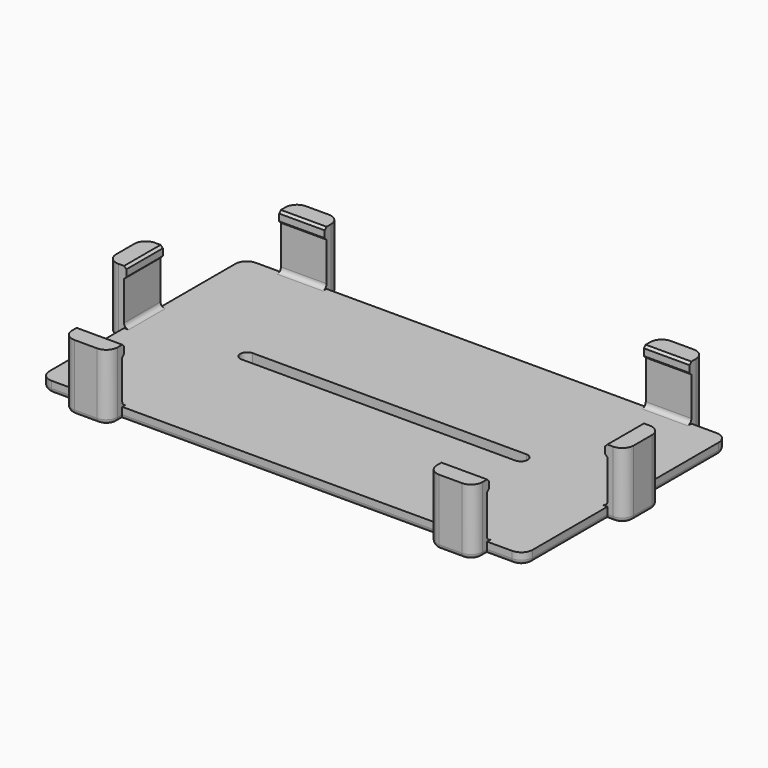
from build123d import *

# Parameters (mm, degrees)
F1_DEPTH = 3.175
F3_DEPTH = 15.24
F4_W     = 1.27
F4_H     = 12.7
F4_W_2   = 12.7
F4_H_2   = 1.27
F5_DEPTH = 3.175
F6_SIZE  = 1.26999
F8_W     = 133.35
F8_H     = 69.85
F9_DEPTH = 6.35
F10_R    = 1.27
F11_R    = 1.27


# Not quite as in the source:
# - a fillet or chamfer is up to 0.001 mm smaller than in the source, because OpenCascade refuses the exact size


with BuildPart() as f1:
    # F0 (on Top) → F1 (new body)
    with BuildSketch(Plane.XY):
        with BuildLine():
            ThreePointArc((67.31, 32.385), (66.3800640303, 34.6300640303), (64.135, 35.56))
            Line((64.135, 35.56), (-64.135, 35.56))
            ThreePointArc((-64.135, 35.56), (-66.3800640303, 34.6300640303), (-67.31, 32.385))
            Line((-67.31, 32.385), (-67.31, -32.385))
            ThreePointArc((-67.31, -32.385), (-66.3800640303, -34.6300640303), (-64.135, -35.56))
            Line((-64.135, -35.56), (64.135, -35.56))
            ThreePointArc((64.135, -35.56), (66.3800640303, -34.6300640303), (67.31, -32.385))
            Line((67.31, -32.385), (67.31, 32.385))
        make_face()
        with BuildLine():
            Line((38.1, -1.905), (-38.1, -1.905))
            ThreePointArc((-38.1, -1.905), (-40.005, 0), (-38.1, 1.905))
            Line((-38.1, 1.905), (38.1, 1.905))
            ThreePointArc((38.1, 1.905), (40.005, 0), (38.1, -1.905))
        make_face(mode=Mode.SUBTRACT)
    extrude(amount=F1_DEPTH)

    # F2 (on Top) → F3 (join)
    with BuildSketch(Plane.XY):
        with BuildLine():
            Line((-67.31, -6.35), (-67.31, 6.35))
            Line((-67.31, 6.35), (-68.8975, 6.35))
            ThreePointArc((-68.8975, 6.35), (-71.1425640303, 5.4200640303), (-72.0725, 3.175))
            Line((-72.0725, 3.175), (-72.0725, -3.175))
            ThreePointArc((-72.0725, -3.175), (-71.1425640303, -5.4200640303), (-68.8975, -6.35))
            Line((-68.8975, -6.35), (-67.31, -6.35))
        make_face()
        with BuildLine():
            Line((-44.45, -37.1475), (-44.45, -35.56))
            Line((-44.45, -35.56), (-57.15, -35.56))
            Line((-57.15, -35.56), (-57.15, -37.1475))
            ThreePointArc((-57.15, -37.1475), (-56.2200640303, -39.3925640303), (-53.975, -40.3225))
            Line((-53.975, -40.3225), (-47.625, -40.3225))
            ThreePointArc((-47.625, -40.3225), (-45.3799359697, -39.3925640303), (-44.45, -37.1475))
        make_face()
        with BuildLine():
            Line((-57.15, 35.56), (-44.45, 35.56))
            Line((-44.45, 35.56), (-44.45, 37.1475))
            ThreePointArc((-44.45, 37.1475), (-45.3799359697, 39.3925640303), (-47.625, 40.3225))
            Line((-47.625, 40.3225), (-53.975, 40.3225))
            ThreePointArc((-53.975, 40.3225), (-56.2200640303, 39.3925640303), (-57.15, 37.1475))
            Line((-57.15, 37.1475), (-57.15, 35.56))
        make_face()
        with BuildLine():
            Line((57.15, -35.56), (44.45, -35.56))
            Line((44.45, -35.56), (44.45, -37.1475))
            ThreePointArc((44.45, -37.1475), (45.3799359697, -39.3925640303), (47.625, -40.3225))
            Line((47.625, -40.3225), (53.975, -40.3225))
            ThreePointArc((53.975, -40.3225), (56.2200640303, -39.3925640303), (57.15, -37.1475))
            Line((57.15, -37.1475), (57.15, -35.56))
        make_face()
        with BuildLine():
            Line((67.31, 6.35), (67.31, -6.35))
            Line((67.31, -6.35), (68.8975, -6.35))
            ThreePointArc((68.8975, -6.35), (71.1425640303, -5.4200640303), (72.0725, -3.175))
            Line((72.0725, -3.175), (72.0725, 3.175))
            ThreePointArc((72.0725, 3.175), (71.1425640303, 5.4200640303), (68.8975, 6.35))
            Line((68.8975, 6.35), (67.31, 6.35))
        make_face()
        with BuildLine():
            Line((44.45, 35.56), (57.15, 35.56))
            Line((57.15, 35.56), (57.15, 37.1475))
            ThreePointArc((57.15, 37.1475), (56.2200640303, 39.3925640303), (53.975, 40.3225))
            Line((53.975, 40.3225), (47.625, 40.3225))
            ThreePointArc((47.625, 40.3225), (45.3799359697, 39.3925640303), (44.45, 37.1475))
            Line((44.45, 37.1475), (44.45, 35.56))
        make_face()
    extrude(amount=F3_DEPTH)

    # F4 (on face) → F5 (join)
    with BuildSketch(Plane.XY.offset(15.24)):
        with BuildLine():
            Line((-68.8975, -6.35), (-67.31, -6.35))
            Line((-67.31, -6.35), (-67.31, 6.35))
            Line((-67.31, 6.35), (-68.8975, 6.35))
            ThreePointArc((-68.8975, 6.35), (-71.1425640303, 5.4200640303), (-72.0725, 3.175))
            Line((-72.0725, 3.175), (-72.0725, -3.175))
            ThreePointArc((-72.0725, -3.175), (-71.1425640303, -5.4200640303), (-68.8975, -6.35))
        make_face()
        with Locations((-66.675, 0)):
            Rectangle(F4_W, F4_H)
        with BuildLine():
            Line((-44.45, -35.56), (-57.15, -35.56))
            Line((-57.15, -35.56), (-57.15, -37.1475))
            ThreePointArc((-57.15, -37.1475), (-56.2200640303, -39.3925640303), (-53.975, -40.3225))
            Line((-53.975, -40.3225), (-47.625, -40.3225))
            ThreePointArc((-47.625, -40.3225), (-45.3799359697, -39.3925640303), (-44.45, -37.1475))
            Line((-44.45, -37.1475), (-44.45, -35.56))
        make_face()
        with Locations((-50.8, -34.925)):
            Rectangle(F4_W_2, F4_H_2)
        with BuildLine():
            Line((-57.15, 37.1475), (-57.15, 35.56))
            Line((-57.15, 35.56), (-44.45, 35.56))
            Line((-44.45, 35.56), (-44.45, 37.1475))
            ThreePointArc((-44.45, 37.1475), (-45.3799359697, 39.3925640303), (-47.625, 40.3225))
            Line((-47.625, 40.3225), (-53.975, 40.3225))
            ThreePointArc((-53.975, 40.3225), (-56.2200640303, 39.3925640303), (-57.15, 37.1475))
        make_face()
        with Locations((-50.8, 34.925)):
            Rectangle(F4_W_2, F4_H_2)
        with Locations((50.8, 34.925)):
            Rectangle(F4_W_2, F4_H_2)
        with BuildLine():
            Line((44.45, 35.56), (57.15, 35.56))
            Line((57.15, 35.56), (57.15, 37.1475))
            ThreePointArc((57.15, 37.1475), (56.2200640303, 39.3925640303), (53.975, 40.3225))
            Line((53.975, 40.3225), (47.625, 40.3225))
            ThreePointArc((47.625, 40.3225), (45.3799359697, 39.3925640303), (44.45, 37.1475))
            Line((44.45, 37.1475), (44.45, 35.56))
        make_face()
        with Locations((66.675, 0)):
            Rectangle(F4_W, F4_H)
        with BuildLine():
            Line((68.8975, 6.35), (67.31, 6.35))
            Line((67.31, 6.35), (67.31, -6.35))
            Line((67.31, -6.35), (68.8975, -6.35))
            ThreePointArc((68.8975, -6.35), (71.1425640303, -5.4200640303), (72.0725, -3.175))
            Line((72.0725, -3.175), (72.0725, 3.175))
            ThreePointArc((72.0725, 3.175), (71.1425640303, 5.4200640303), (68.8975, 6.35))
        make_face()
        with BuildLine():
            Line((57.15, -37.1475), (57.15, -35.56))
            Line((57.15, -35.56), (44.45, -35.56))
            Line((44.45, -35.56), (44.45, -37.1475))
            ThreePointArc((44.45, -37.1475), (45.3799359697, -39.3925640303), (47.625, -40.3225))
            Line((47.625, -40.3225), (53.975, -40.3225))
            ThreePointArc((53.975, -40.3225), (56.2200640303, -39.3925640303), (57.15, -37.1475))
        make_face()
        with Locations((50.8, -34.925)):
            Rectangle(F4_W_2, F4_H_2)
    extrude(amount=F5_DEPTH)

    # F6 (size 1.27 in the source; OpenCascade refuses exactly that, so slightly less here)
    f6_edges = [f1.edges().sort_by_distance(p)[0] for p in [
        (50.8, -34.29, 15.24),
        (50.8, -34.29, 18.415),
        (66.04, 0, 18.415),
        (50.8, 34.29, 18.415),
        (-50.8, -34.29, 18.415),
        (-66.04, 0, 18.415),
        (-50.8, 34.29, 18.415),
        (-66.04, 0, 15.24),
        (-50.8, -34.29, 15.24),
        (66.04, 0, 15.24),
        (50.8, 34.29, 15.24),
        (-50.8, 34.29, 15.24),
    ]]
    chamfer(f6_edges, length=F6_SIZE)

    # F8 (on face) → F9 (cut)
    with BuildSketch(Plane.XY.offset(18.415)):
        Rectangle(F8_W, F8_H)
    extrude(amount=-F9_DEPTH, mode=Mode.SUBTRACT)

    # F10
    f10_edges = [f1.edges().sort_by_distance(p)[0] for p in [
        (-50.8, -40.3225, 0),
        (-45.379936, -39.392564, 0),
        (-56.220064, -39.392564, 0),
        (0, -35.56, 0),
        (45.379936, -39.392564, 0),
        (56.220064, -39.392564, 0),
        (60.6425, -35.56, 0),
        (71.142564, -5.420064, 0),
        (67.31, 19.3675, 0),
        (56.220064, 39.392564, 0),
        (0, 35.56, 0),
        (-50.8, 40.3225, 0),
        (-60.6425, 35.56, 0),
        (-71.142564, 5.420064, 0),
        (-67.31, -19.3675, 0),
    ]]
    fillet(f10_edges, radius=F10_R)

    # F11
    f11_edges = [f1.edges().sort_by_distance(p)[0] for p in [
        (67.31, 0, 3.175),
        (-50.8, -35.56, 3.175),
        (50.8, -35.56, 3.175),
        (-67.31, 0, 3.175),
        (50.8, 35.56, 3.175),
        (-50.8, 35.56, 3.175),
    ]]
    fillet(f11_edges, radius=F11_R)


solid = f1.part
